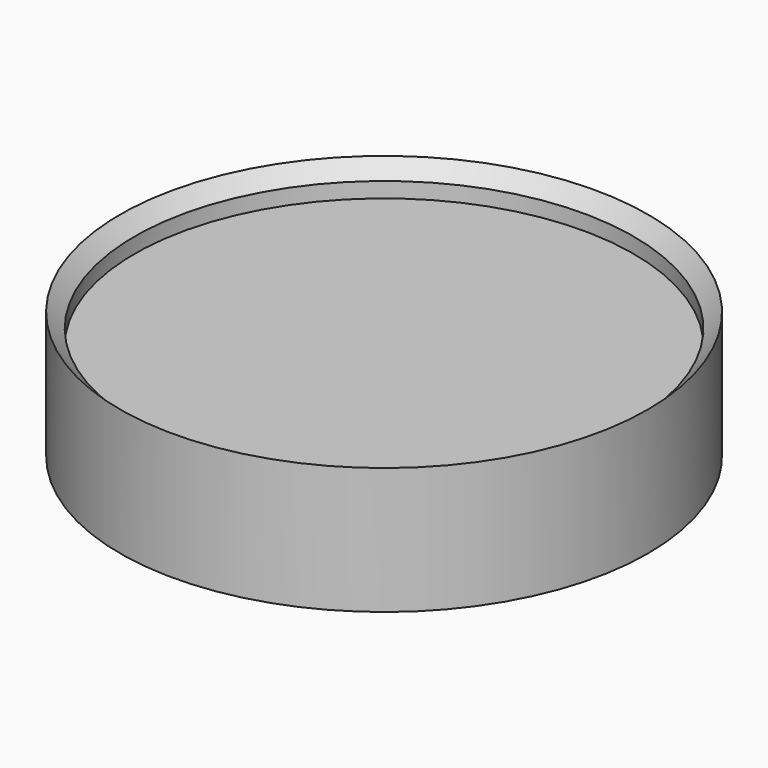
from build123d import *

# Parameters (mm, degrees)
F0_R     = 13.1445
F1_DEPTH = 4.826
F2_R     = 13.1445
F2_R_2   = 12.4206
F3_DEPTH = 1.524


# Not quite as in the source:
# - a fillet or chamfer that OpenCascade refuses, or shapes differently, is made with other operations: its cross-section is extruded or revolved along the edge and cut away or added


with BuildPart() as f1:
    # F0 (on Top) → F1 (new body)
    with BuildSketch(Plane.XY):
        Circle(F0_R)
    extrude(amount=F1_DEPTH)

    # F2 (on face) → F3 (join)
    with BuildSketch(Plane.XY.offset(4.826)):
        Circle(F2_R)
        Circle(F2_R_2, mode=Mode.SUBTRACT)
    extrude(amount=F3_DEPTH)

    # F4: chamfer of 0.762 on 1 edges, made by hand

    # F4_s1 → F4_t2 (revolve, cut)
    with BuildSketch(Plane.XZ):
        Polygon((13.1826, 6.35), (12.4206, 5.588), (12.4206, 6.35), align=None)
    revolve(axis=Axis((0, 0, 6.35), (0, 0, 1)), mode=Mode.SUBTRACT)


solid = f1.part
